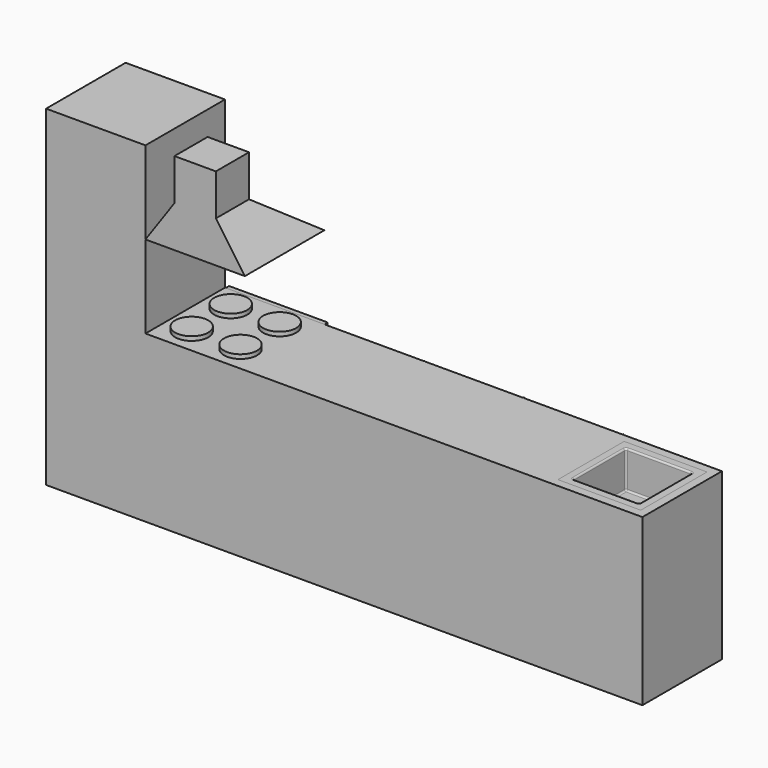
from build123d import *

# Parameters (mm, degrees)
F0_W       = 3600
F0_H       = 600
F1_DEPTH   = 1000
F2_W       = 500
F2_H       = 500
F3_DEPTH   = 250
F4_W       = 500
F4_H       = 500
F5_DEPTH   = 25
F6_W       = 500
F6_H       = 500
F6_W_2     = 400
F6_H_2     = 400
F7_DEPTH   = 225
F8_R       = 10
F9_R       = 12.8028507665
F10_DEPTH  = 25
F11_W      = 5
F11_H      = 1000
F11_R      = 25
F12_DEPTH  = 5
F13_R      = 100
F14_DEPTH  = 25
F15_W      = 595
F15_H      = 150
F16_DEPTH  = 25
F15_H_2    = 800
F17_W      = 495
F17_H      = 495
F18_DEPTH  = 5
F17_R      = 40
F19_W      = 600
F19_H      = 600
F20_DEPTH  = 1000
F21_W      = 600
F21_H      = 10
F22_DEPTH  = 50
F24_DEPTH  = 25
F25_W      = 250
F25_H      = 250
F26_DEPTH  = 250
F26_FACE_W = 250
F26_FACE_H = 250
F28_W      = 600
F28_H      = 600


with BuildPart() as f1:
    # F0 (on Top) → F1 (new body)
    with BuildSketch(Plane.XY):
        with Locations((1800, 300)):
            Rectangle(F0_W, F0_H)
    extrude(amount=F1_DEPTH)

    # F2 (on face) → F3 (cut)
    with BuildSketch(Plane.XY.offset(1000)):
        with Locations((3300, 300)):
            Rectangle(F2_W, F2_H)
    extrude(amount=-F3_DEPTH, mode=Mode.SUBTRACT)

    # F11 (on face) → F12 (join)
    with BuildSketch(Plane(origin=(0, 600, 0), x_dir=(-1, 0, 0), z_dir=(0, 1, 0))):
        with Locations((-3002.5, 500)):
            Rectangle(F11_W, F11_H)
        with Locations((-2402.5, 500)):
            Rectangle(F11_W, F11_H)
        with Locations((-1802.5, 500)):
            Rectangle(F11_W, F11_H)
        with Locations((-1202.5, 500)):
            Rectangle(F11_W, F11_H)
        with Locations((-602.5, 500)):
            Rectangle(F11_W, F11_H)
        with Locations((-3075, 500)):
            Circle(F11_R)
        with Locations((-2930, 500)):
            Circle(F11_R)
        with Locations((-1730, 500)):
            Circle(F11_R)
        with Locations((-1875, 500)):
            Circle(F11_R)
    extrude(amount=F12_DEPTH)

    # F19 (on face) → F20 (join)
    with BuildSketch(Plane.XY.offset(1000)):
        with Locations((300, 300)):
            Rectangle(F19_W, F19_H)
    extrude(amount=F20_DEPTH)

    # F21 (on face) → F22 (cut)
    with BuildSketch(Plane(origin=(0, 600, 0), x_dir=(-1, 0, 0), z_dir=(0, 1, 0))):
        with Locations((-300, 1545)):
            Rectangle(F21_W, F21_H)
    extrude(amount=-F22_DEPTH, mode=Mode.SUBTRACT)

    # F23 (on face) → F24 (join)
    with BuildSketch(Plane(origin=(0, 600, 0), x_dir=(-1, 0, 0), z_dir=(0, 1, 0))):
        with BuildLine():
            Line((-550, 1850), (-550, 1775))
            Line((-550, 1775), (-550, 1700))
            ThreePointArc((-550, 1700), (-540, 1690), (-530, 1700))
            Line((-530, 1700), (-530, 1775))
            Line((-530, 1775), (-530, 1850))
            ThreePointArc((-530, 1850), (-540, 1860), (-550, 1850))
        make_face()
        with BuildLine():
            Line((-550, 1324.8867511749), (-550, 1249.8867511749))
            Line((-550, 1249.8867511749), (-550, 1174.8867511749))
            ThreePointArc((-550, 1174.8867511749), (-540, 1164.8867511749), (-530, 1174.8867511749))
            Line((-530, 1174.8867511749), (-530, 1249.8867511749))
            Line((-530, 1249.8867511749), (-530, 1324.8867511749))
            ThreePointArc((-530, 1324.8867511749), (-540, 1334.8867511749), (-550, 1324.8867511749))
        make_face()
    extrude(amount=F24_DEPTH)


with BuildPart() as f5:
    # F4 (on face) → F5 (new body)
    with BuildSketch(Plane.XY.offset(750)):
        with Locations((3300, 300)):
            Rectangle(F4_W, F4_H)
    extrude(amount=F5_DEPTH)

    # F6 (on face) → F7 (join, through all)
    with BuildSketch(Plane.XY.offset(775)):
        with Locations((3300, 300)):
            Rectangle(F6_W, F6_H)
        with Locations((3300, 300)):
            Rectangle(F6_W_2, F6_H_2, mode=Mode.SUBTRACT)
    extrude(amount=F7_DEPTH)

    # F8
    f8_edges = [f5.edges().sort_by_distance(p)[0] for p in [
        (3500, 300, 1000),
        (3300, 500, 1000),
        (3100, 300, 1000),
        (3300, 100, 1000),
        (3500, 500, 887.5),
        (3300, 500, 775),
        (3500, 300, 775),
        (3300, 100, 775),
        (3500, 100, 887.5),
        (3100, 100, 887.5),
        (3100, 300, 775),
        (3100, 500, 887.5),
    ]]
    fillet(f8_edges, radius=F8_R)

    # F9 (on face) → F10 (cut)
    with BuildSketch(Plane.XY.offset(775)):
        with Locations((3300, 143.9911872149)):
            Circle(F9_R)
    extrude(amount=-F10_DEPTH, mode=Mode.SUBTRACT)


with BuildPart() as f14:
    # F13 (on face) → F14 (new body)
    with BuildSketch(Plane.XY.offset(1000)):
        with Locations((1050, 155)):
            Circle(F13_R)
    extrude(amount=F14_DEPTH)


with BuildPart() as f14b:
    # F13 (on face) → F14, piece 2 (new body)
    with BuildSketch(Plane.XY.offset(1000)):
        with Locations((755, 155)):
            Circle(F13_R)
    extrude(amount=F14_DEPTH)


with BuildPart() as f14c:
    # F13 (on face) → F14, piece 3 (new body)
    with BuildSketch(Plane.XY.offset(1000)):
        with Locations((755, 450)):
            Circle(F13_R)
    extrude(amount=F14_DEPTH)


with BuildPart() as f14d:
    # F13 (on face) → F14, piece 4 (new body)
    with BuildSketch(Plane.XY.offset(1000)):
        with Locations((1050, 450)):
            Circle(F13_R)
    extrude(amount=F14_DEPTH)


with BuildPart() as f16:
    # F15 (on face) → F16 (new body)
    with BuildSketch(Plane(origin=(0, 600, 0), x_dir=(-1, 0, 0), z_dir=(0, 1, 0))):
        with Locations((-902.5, 925)):
            Rectangle(F15_W, F15_H)
    extrude(amount=F16_DEPTH)


with BuildPart() as f16b:
    # F15 (on face) → F16, piece 2 (new body)
    with BuildSketch(Plane(origin=(0, 600, 0), x_dir=(-1, 0, 0), z_dir=(0, 1, 0))):
        with Locations((-902.5, 445)):
            Rectangle(F15_W, F15_H_2)
    extrude(amount=F16_DEPTH)


with BuildPart() as f18:
    # F17 (on face) → F18 (new body)
    with BuildSketch(Plane(origin=(0, 625, 0), x_dir=(-1, 0, 0), z_dir=(0, 1, 0))):
        with Locations((-902.5, 497.5)):
            Rectangle(F17_W, F17_H)
    extrude(amount=F18_DEPTH)


with BuildPart() as f18b:
    # F17 (on face) → F18, piece 2 (new body)
    with BuildSketch(Plane(origin=(0, 625, 0), x_dir=(-1, 0, 0), z_dir=(0, 1, 0))):
        with Locations((-753.75, 925)):
            Circle(F17_R)
    extrude(amount=F18_DEPTH)


with BuildPart() as f18c:
    # F17 (on face) → F18, piece 3 (new body)
    with BuildSketch(Plane(origin=(0, 625, 0), x_dir=(-1, 0, 0), z_dir=(0, 1, 0))):
        with Locations((-1051.25, 925)):
            Circle(F17_R)
    extrude(amount=F18_DEPTH)


with BuildPart() as f26:
    # F25 (on face) → F26 (new body)
    with BuildSketch(Plane.XY.offset(2000)):
        with Locations((900, 125)):
            Rectangle(F25_W, F25_H)
    extrude(amount=-F26_DEPTH)

    # F26_face (on face) → F29 section 0
    with BuildSketch(Plane(origin=(900, 125, 1750), x_dir=(1, 0, 0), z_dir=(0, 0, -1))):
        Rectangle(F26_FACE_W, F26_FACE_H)
    # F28 (on offset) → F29 section 1
    with BuildSketch(Plane(origin=(0, 0, 1500), x_dir=(1, 0, 0), z_dir=(0, 0, -1))):
        with Locations((900, -300)):
            Rectangle(F28_W, F28_H)
    loft()


solid = Compound([f1.part, f5.part, f14.part, f14b.part, f14c.part, f14d.part, f16.part, f16b.part, f18.part, f18b.part, f18c.part, f26.part])
